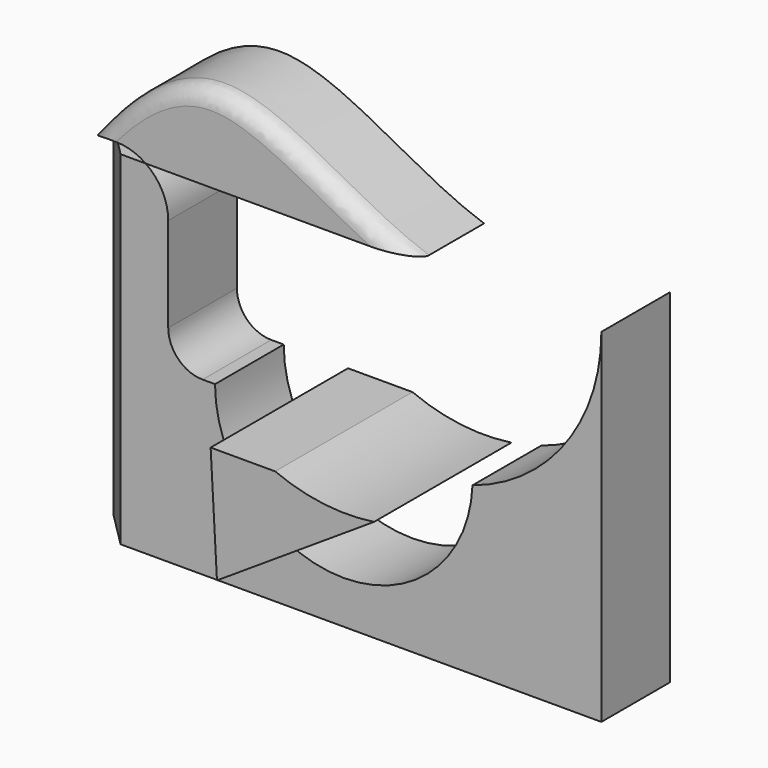
from build123d import *

# Parameters (mm, degrees)
F1_DEPTH = 12.7
F2_DEPTH = 25.4
F3_R     = 2.54
F5_SIZE  = 5.08
F6_R     = 5.08


# Not quite as in the source:
# - a feature of the source that left no trace in its solid (it failed there, or was rolled back) is left out


with BuildPart() as f1:
    # F0 (on Front) → F1 (new body)
    with BuildSketch(Plane.XZ):
        with BuildLine():
            ThreePointArc((14.6395320428, -1.8160650439), (7.1957981438, -1.9073534013), (0, 0))
            Line((0, 0), (-9.5393729797, 0))
            Line((-9.5393729797, 0), (-8.6053529899, -16.9955994281))
            Line((-8.6053529899, -16.9955994281), (14.6395320428, -1.8160650439))
        make_face()
    extrude(amount=-F1_DEPTH)

    # F2 (add): a face of the model
    f2_faces = [f1.faces().sort_by_distance(p)[0] for p in [
        (-1.4587062215, 12.7, -6.2717912086),
    ]]


with BuildPart() as f1b:
    # F0 (on Front) → F1, piece 2 (new body)
    with BuildSketch(Plane.XZ):
        with BuildLine():
            ThreePointArc((-8.6053529899, -16.9955994281), (-16.2301336171, -9.9742299338), (-19.05, 0))
            Line((-19.05, 0), (-25.971364924, 0))
            Line((-25.971364924, 0), (-25.971364924, 19.05))
            ThreePointArc((-25.971364924, 19.05), (-26.8527815535, 22.633827134), (-29.2959352279, 25.4))
            Line((-29.2959352279, 25.4), (-38.1, 25.4))
            Line((-38.1, 25.4), (-38.1, -25.4))
            Line((-38.1, -25.4), (38.1, -25.4))
            Line((38.1, -25.4), (38.1, 25.4))
            ThreePointArc((38.1, 25.4), (32.8284890456, 9.2037043809), (19.0337377265, -0.7869740527))
            ThreePointArc((19.0337377265, -0.7869740527), (9.6367881679, -16.4327360414), (-8.6053529899, -16.9955994281))
        make_face()
    extrude(amount=-F1_DEPTH)


with BuildPart() as f1c:
    # F0 (on Front) → F1, piece 3 (new body)
    with BuildSketch(Plane.XZ):
        with BuildLine():
            ThreePointArc((-38.1, 25.4), (-33.6979676139, 26.7766026899), (-29.2959352279, 25.4))
            Line((-29.2959352279, 25.4), (10.5833333333, 25.4))
            add(Edge.make_bspline(
                [(-38.1, 25.4), (-32.4034356926, 32.7258786812), (-19.1819964183, 44.9419170764), (0.319873071, 28.826665029), (10.5833333333, 25.4)],
                knots=[0, 0, 0, 0, 0.304709608, 0.6658251219, 0.6658251219, 0.6658251219, 0.6658251219], degree=3))
        make_face()
    extrude(amount=-F1_DEPTH)

    # F3
    f3_edges = [f1c.edges().sort_by_distance(p)[0] for p in [
        (-14.799697, 0, 37.233797),
    ]]
    fillet(f3_edges, radius=F3_R)


with BuildPart() as f1_1:
    add(f1.part)

    add(f1b.part)  # F2 merges F1b
    extrude(f2_faces, amount=-F2_DEPTH)

    # F5
    f5_edges = [f1_1.edges().sort_by_distance(p)[0] for p in [
        (-38.1, 0, 0),
    ]]
    chamfer(f5_edges, length=F5_SIZE)

    # F6
    f6_edges = [f1_1.edges().sort_by_distance(p)[0] for p in [
        (-25.971365, 6.35, 0),
    ]]
    fillet(f6_edges, radius=F6_R)


solid = Compound([f1c.part, f1_1.part])
